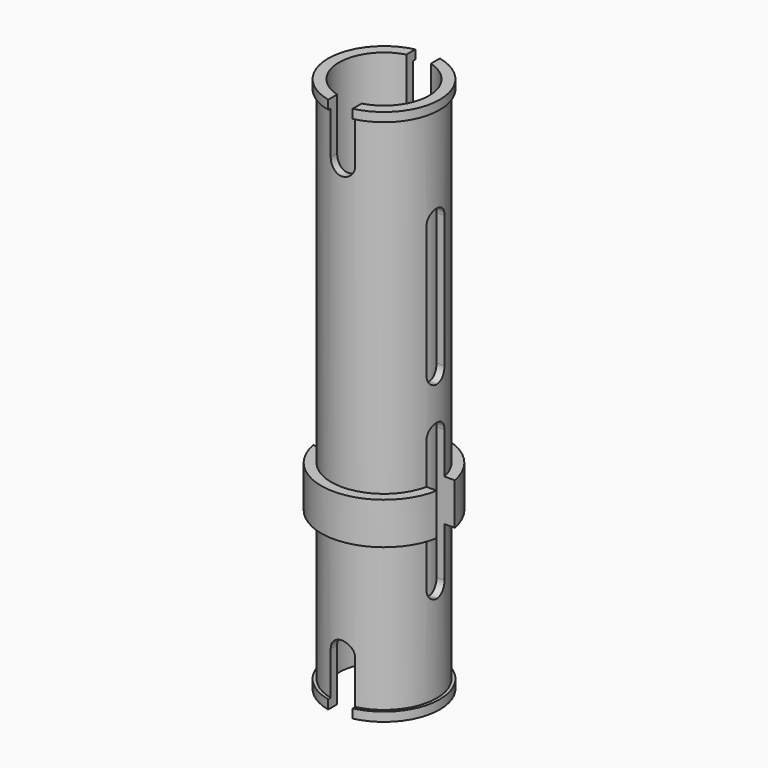
from build123d import *

# Parameters (mm, degrees)
F0_R      = 2.345
F1_DEPTH  = 11.94
F2_DEPTH  = 11.94
F5_DEPTH  = 166.5
F6_DEPTH  = 12.5
F7_W      = 0.5
F7_H      = 1.86
F4_W      = 1
F4_H      = 6.89
F9_DEPTH  = 12.5
F10_R     = 2
F11_DEPTH = 20.5
F12_W     = 0.2
F12_H     = 0.4
F14_DEPTH = 12.5
F15_DEPTH = 25
F16_DEPTH = 12.5
F17_R     = 0.4999


# Not quite as in the source:
# - a fillet or chamfer is up to 0.001 mm smaller than in the source, because OpenCascade refuses the exact size
# - a pattern or mirror of a feature is missing from the dataset's text; its kind, count and spacing are read off the source's solid


with BuildPart() as f1:
    # F0 (on Top) → F1 (new body)
    with BuildSketch(Plane.XY):
        Circle(F0_R)
    extrude(amount=F1_DEPTH)

    # F0 (on Top) → F2 (join)
    with BuildSketch(Plane.XY):
        Circle(F0_R)
    extrude(amount=-F2_DEPTH)

    # F3 (on Front) → F5 (cut, symmetric)
    with BuildSketch(Plane.XZ):
        with BuildLine():
            Line((-0.545, -12.9641438561), (0.545, -12.9641438561))
            Line((0.545, -12.9641438561), (0.545, -9.629))
            ThreePointArc((0.545, -9.629), (0, -10.174), (-0.545, -9.629))
            Line((-0.545, -9.629), (-0.545, -12.9641438561))
        make_face()
        with BuildLine():
            ThreePointArc((-0.545, -9.629), (0, -10.174), (0.545, -9.629))
            Line((0.545, -9.629), (-0.545, -9.629))
        make_face()
        with BuildLine():
            Line((-0.545, -9.629), (0.545, -9.629))
            ThreePointArc((0.545, -9.629), (0, -9.084), (-0.545, -9.629))
        make_face()
        with BuildLine():
            ThreePointArc((-0.545, 9.629), (0, 9.084), (0.545, 9.629))
            ThreePointArc((0.545, 9.629), (0, 10.174), (-0.545, 9.629))
        make_face()
        with BuildLine():
            ThreePointArc((-0.545, 9.629), (0, 10.174), (0.545, 9.629))
            Line((0.545, 9.629), (0.545, 12.9641438561))
            Line((0.545, 12.9641438561), (-0.545, 12.9641438561))
            Line((-0.545, 12.9641438561), (-0.545, 9.629))
        make_face()
    extrude(amount=F5_DEPTH, both=True, mode=Mode.SUBTRACT)

    # F3 (on Front) → F6 (cut, symmetric)
    with BuildSketch(Plane.XZ):
        with BuildLine():
            Line((-0.545, -12.9641438561), (0.545, -12.9641438561))
            Line((0.545, -12.9641438561), (0.545, -9.629))
            ThreePointArc((0.545, -9.629), (0, -10.174), (-0.545, -9.629))
            Line((-0.545, -9.629), (-0.545, -12.9641438561))
        make_face()
        with BuildLine():
            ThreePointArc((-0.545, -9.629), (0, -10.174), (0.545, -9.629))
            Line((0.545, -9.629), (-0.545, -9.629))
        make_face()
        with BuildLine():
            Line((-0.545, -9.629), (0.545, -9.629))
            ThreePointArc((0.545, -9.629), (0, -9.084), (-0.545, -9.629))
        make_face()
        with BuildLine():
            ThreePointArc((-0.545, 9.629), (0, 9.084), (0.545, 9.629))
            ThreePointArc((0.545, 9.629), (0, 10.174), (-0.545, 9.629))
        make_face()
        with BuildLine():
            ThreePointArc((-0.545, 9.629), (0, 10.174), (0.545, 9.629))
            Line((0.545, 9.629), (0.545, 12.9641438561))
            Line((0.545, 12.9641438561), (-0.545, 12.9641438561))
            Line((-0.545, 12.9641438561), (-0.545, 9.629))
        make_face()
    extrude(amount=F6_DEPTH, both=True, mode=Mode.SUBTRACT)

    # F7 (on Front) → F8 (revolve)
    with BuildSketch(Plane.XZ):
        with Locations((-2.5410750752, -4.01)):
            Rectangle(F7_W, F7_H)
    revolve(axis=Axis((0, 0, 0), (0, 0, -1)))

    # F4 (on Right) → F9 (cut, symmetric)
    with BuildSketch(Plane.YZ):
        with Locations((0, -4.195)):
            Rectangle(F4_W, F4_H)
        with Locations((0, 4.195)):
            Rectangle(F4_W, F4_H)
    extrude(amount=F9_DEPTH, both=True, mode=Mode.SUBTRACT)

    # F10 (on Top) → F11 (cut, symmetric)
    with BuildSketch(Plane.XY):
        Circle(F10_R)
    extrude(amount=F11_DEPTH, both=True, mode=Mode.SUBTRACT)

    # F12 (on Right) → F13 (revolve)
    with BuildSketch(Plane.YZ):
        with Locations((2.380789337, 11.74)):
            Rectangle(F12_W, F12_H)
    f13 = revolve(axis=Axis((0, 0, 0), (0, 0, -1)))

    # F13_copies: F13 across plane
    add(f13.mirror(Plane(origin=(0, 0, 0), x_dir=(-1, 0, 0), z_dir=(0, 0, -1))))

    # F3 (on Front) → F14 (cut, symmetric)
    with BuildSketch(Plane.XZ):
        with BuildLine():
            Line((-0.545, -12.9641438561), (0.545, -12.9641438561))
            Line((0.545, -12.9641438561), (0.545, -9.629))
            ThreePointArc((0.545, -9.629), (0, -10.174), (-0.545, -9.629))
            Line((-0.545, -9.629), (-0.545, -12.9641438561))
        make_face()
        with BuildLine():
            ThreePointArc((-0.545, -9.629), (0, -10.174), (0.545, -9.629))
            Line((0.545, -9.629), (-0.545, -9.629))
        make_face()
        with BuildLine():
            Line((-0.545, -9.629), (0.545, -9.629))
            ThreePointArc((0.545, -9.629), (0, -9.084), (-0.545, -9.629))
        make_face()
        with BuildLine():
            ThreePointArc((-0.545, 9.629), (0, 9.084), (0.545, 9.629))
            ThreePointArc((0.545, 9.629), (0, 10.174), (-0.545, 9.629))
        make_face()
        with BuildLine():
            ThreePointArc((-0.545, 9.629), (0, 10.174), (0.545, 9.629))
            Line((0.545, 9.629), (0.545, 12.9641438561))
            Line((0.545, 12.9641438561), (-0.545, 12.9641438561))
            Line((-0.545, 12.9641438561), (-0.545, 9.629))
        make_face()
    extrude(amount=F14_DEPTH, both=True, mode=Mode.SUBTRACT)

    # F3 (on Front) → F15 (cut)
    with BuildSketch(Plane.XZ):
        with BuildLine():
            Line((-0.545, -12.9641438561), (0.545, -12.9641438561))
            Line((0.545, -12.9641438561), (0.545, -9.629))
            ThreePointArc((0.545, -9.629), (0, -10.174), (-0.545, -9.629))
            Line((-0.545, -9.629), (-0.545, -12.9641438561))
        make_face()
        with BuildLine():
            ThreePointArc((-0.545, -9.629), (0, -10.174), (0.545, -9.629))
            Line((0.545, -9.629), (-0.545, -9.629))
        make_face()
        with BuildLine():
            Line((-0.545, -9.629), (0.545, -9.629))
            ThreePointArc((0.545, -9.629), (0, -9.084), (-0.545, -9.629))
        make_face()
        with BuildLine():
            ThreePointArc((-0.545, 9.629), (0, 9.084), (0.545, 9.629))
            ThreePointArc((0.545, 9.629), (0, 10.174), (-0.545, 9.629))
        make_face()
        with BuildLine():
            ThreePointArc((-0.545, 9.629), (0, 10.174), (0.545, 9.629))
            Line((0.545, 9.629), (0.545, 12.9641438561))
            Line((0.545, 12.9641438561), (-0.545, 12.9641438561))
            Line((-0.545, 12.9641438561), (-0.545, 9.629))
        make_face()
    extrude(amount=-F15_DEPTH, mode=Mode.SUBTRACT)

    # F3 (on Front) → F16 (cut, symmetric)
    with BuildSketch(Plane.XZ):
        with BuildLine():
            Line((-0.545, -12.9641438561), (0.545, -12.9641438561))
            Line((0.545, -12.9641438561), (0.545, -9.629))
            ThreePointArc((0.545, -9.629), (0, -10.174), (-0.545, -9.629))
            Line((-0.545, -9.629), (-0.545, -12.9641438561))
        make_face()
        with BuildLine():
            ThreePointArc((-0.545, -9.629), (0, -10.174), (0.545, -9.629))
            Line((0.545, -9.629), (-0.545, -9.629))
        make_face()
        with BuildLine():
            Line((-0.545, -9.629), (0.545, -9.629))
            ThreePointArc((0.545, -9.629), (0, -9.084), (-0.545, -9.629))
        make_face()
        with BuildLine():
            ThreePointArc((-0.545, 9.629), (0, 9.084), (0.545, 9.629))
            ThreePointArc((0.545, 9.629), (0, 10.174), (-0.545, 9.629))
        make_face()
        with BuildLine():
            ThreePointArc((-0.545, 9.629), (0, 10.174), (0.545, 9.629))
            Line((0.545, 9.629), (0.545, 12.9641438561))
            Line((0.545, 12.9641438561), (-0.545, 12.9641438561))
            Line((-0.545, 12.9641438561), (-0.545, 9.629))
        make_face()
    extrude(amount=F16_DEPTH, both=True, mode=Mode.SUBTRACT)

    # F17 (radius 0.5 in the source; OpenCascade refuses exactly that, so slightly less here)
    f17_edges = [f1.edges().sort_by_distance(p)[0] for p in [
        (2.113783, 0.5, 0.75),
        (-2.113783, 0.5, 0.75),
        (2.113783, -0.5, 0.75),
        (-2.113783, -0.5, 0.75),
        (2.113783, -0.5, -0.75),
        (-2.113783, -0.5, -0.75),
        (2.113783, 0.5, -0.75),
        (-2.113783, 0.5, -0.75),
        (-2.113783, -0.5, -7.64),
        (2.113783, -0.5, -7.64),
        (2.113783, 0.5, -7.64),
        (-2.113783, 0.5, -7.64),
        (2.113783, -0.5, 7.64),
        (-2.113783, -0.5, 7.64),
        (2.113783, 0.5, 7.64),
        (-2.113783, 0.5, 7.64),
    ]]
    fillet(f17_edges, radius=F17_R)


solid = f1.part
